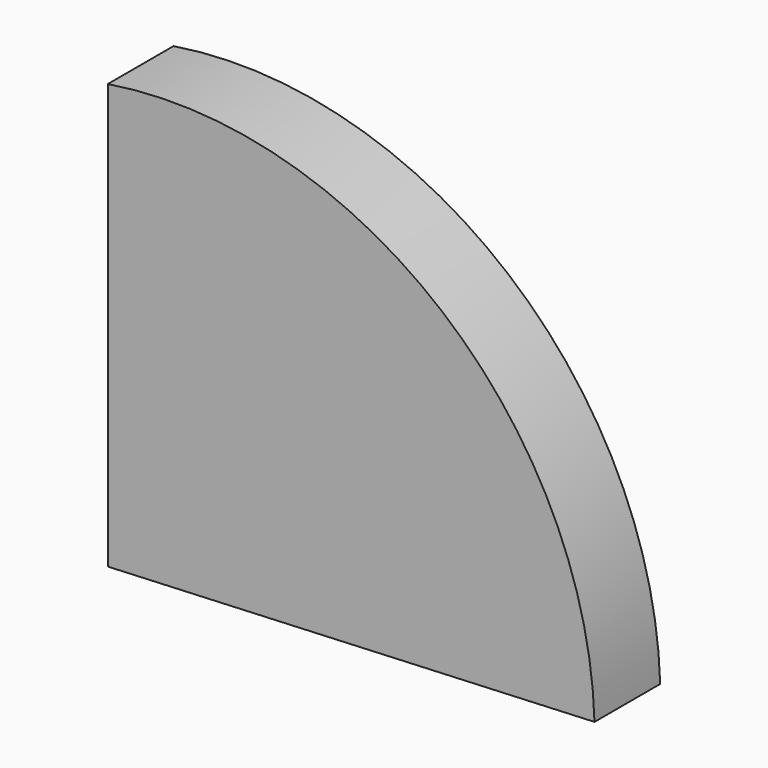
from build123d import *

# Parameters (mm, degrees)
F1_DEPTH    = 25.4
F2_T1_DEPTH = 811.0633942267


# Not quite as in the source:
# - a fillet or chamfer that OpenCascade refuses, or shapes differently, is made with other operations: its cross-section is extruded or revolved along the edge and cut away or added


with BuildPart() as f1:
    # F0 (on Front) → F1 (new body)
    with BuildSketch(Plane.XZ):
        Polygon((0, 131.385833025), (0, 0), (150.5763530731, 6.660095416), (150.5763530731, 159.9298715591), align=None)
    extrude(amount=F1_DEPTH)

    # F2: fillet of radius 130.1940036456 on 1 edges, made by hand

    # F2_s2 → F2_t1 (cut)
    with BuildSketch(Plane.XZ.offset(-392.8316971133)):
        with BuildLine():
            ThreePointArc((150.5763530731, 2.7971927138), (104.9306164399, 101.8025922154), (0, 131.385833025))
            Line((0, 131.385833025), (-0.4076469886, 133.9576058312))
            ThreePointArc((-0.4076469886, 133.9576058312), (74.8032082099, 148.2161714974), (150.0913847465, 162.4881907645))
            Line((150.0913847465, 162.4881907645), (153.180233146, 159.9298715591))
            Line((153.180233146, 159.9298715591), (153.180233146, 2.7971927138))
            Line((153.180233146, 2.7971927138), (150.5763530731, 2.7971927138))
        make_face()
    extrude(amount=F2_T1_DEPTH, mode=Mode.SUBTRACT)


solid = f1.part
